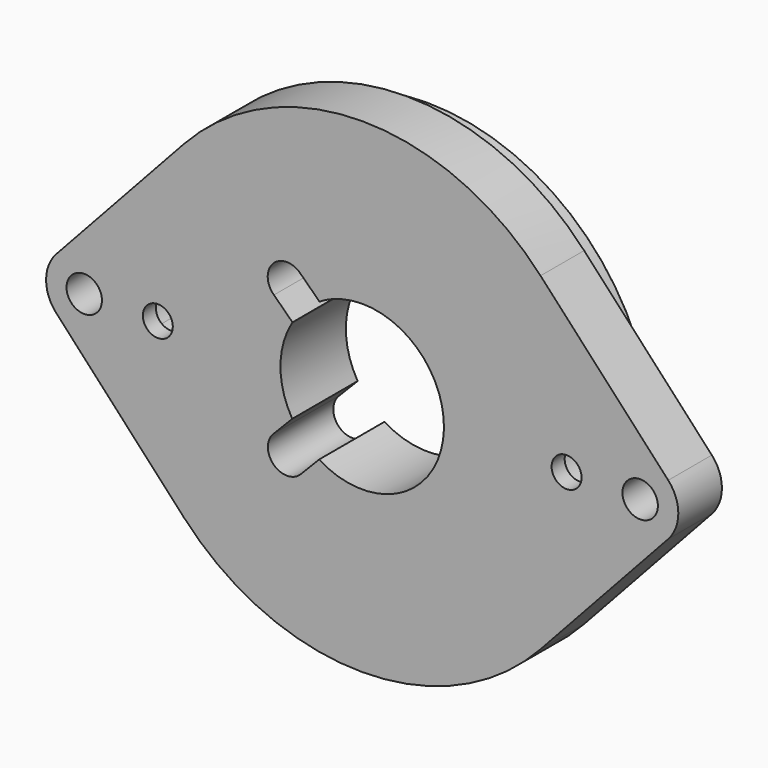
from build123d import *

# Parameters (mm, degrees)
F0_R        = 3.25
F0_R_2      = 41.5
F0_R_3      = 2.75
F1_DEPTH    = 10
F2_DEPTH    = 15
F3_R        = 2.75
F4_DEPTH    = 12
F5_T2_ANGLE = 170.4527374882
F5_T4_ANGLE = 170.4527374882


# Not quite as in the source:
# - a fillet or chamfer that OpenCascade refuses, or shapes differently, is made with other operations: its cross-section is extruded or revolved along the edge and cut away or added


with BuildPart() as f1:
    # F0 (on Front) → F1 (new body)
    with BuildSketch(Plane.XZ):
        with BuildLine():
            Line((56.1470588235, 4.7442370796), (32.7205882353, 30.159792863))
            ThreePointArc((32.7205882353, 30.159792863), (0, 44.5), (-32.7205882353, 30.159792863))
            Line((-32.7205882353, 30.159792863), (-56.1470588235, 4.7442370796))
            ThreePointArc((-56.1470588235, 4.7442370796), (-58, 0), (-56.1470588235, -4.7442370796))
            Line((-56.1470588235, -4.7442370796), (-32.7205882353, -30.159792863))
            ThreePointArc((-32.7205882353, -30.159792863), (0, -44.5), (32.7205882353, -30.159792863))
            Line((32.7205882353, -30.159792863), (56.1470588235, -4.7442370796))
            ThreePointArc((56.1470588235, -4.7442370796), (58, 0), (56.1470588235, 4.7442370796))
        make_face()
        with Locations((-51, 0)):
            Circle(F0_R, mode=Mode.SUBTRACT)
        Circle(F0_R_2, mode=Mode.SUBTRACT)
        with Locations((51, 0)):
            Circle(F0_R, mode=Mode.SUBTRACT)
        Circle(F0_R_2)
        with BuildLine():
            ThreePointArc((-5.5275883623, 13.9443811945), (14.9403084329, -1.336855987), (-7.9154361587, -12.7415018902))
            Line((-7.9154361587, -12.7415018902), (-11.2935258895, -16.2148281895))
            ThreePointArc((-11.2935258895, -16.2148281895), (-16.2431437728, -16.28328537), (-16.3109133443, -11.3336580242))
            Line((-16.3109133443, -11.3336580242), (-12.8354378119, -7.7621863014))
            ThreePointArc((-12.8354378119, -7.7621863014), (-14.9994558699, -0.1277638746), (-12.9658008757, 7.5424139141))
            ThreePointArc((-12.9658008757, 7.5424139141), (-12.8781036996, 7.6911926971), (-12.7886994065, 7.8389519382))
            Line((-12.7886994065, 7.8389519382), (-16.1911722961, 11.1499710909))
            ThreePointArc((-16.1911722961, 11.1499710909), (-16.3869084591, 16.1374875976), (-11.3967981993, 16.2489916113))
            Line((-11.3967981993, 16.2489916113), (-7.8389519382, 12.7886994065))
            ThreePointArc((-7.8389519382, 12.7886994065), (-6.7082039325, 13.416407865), (-5.5275883623, 13.9443811945))
        make_face(mode=Mode.SUBTRACT)
        with Locations((-37.5, 0)):
            Circle(F0_R_3, mode=Mode.SUBTRACT)
        with Locations((37.5, 0)):
            Circle(F0_R_3, mode=Mode.SUBTRACT)
    extrude(amount=-F1_DEPTH)

    # F0 (on Front) → F2 (join)
    with BuildSketch(Plane.XZ):
        Circle(F0_R_2)
        with BuildLine():
            ThreePointArc((-5.5275883623, 13.9443811945), (14.9403084329, -1.336855987), (-7.9154361587, -12.7415018902))
            Line((-7.9154361587, -12.7415018902), (-11.2935258895, -16.2148281895))
            ThreePointArc((-11.2935258895, -16.2148281895), (-16.2431437728, -16.28328537), (-16.3109133443, -11.3336580242))
            Line((-16.3109133443, -11.3336580242), (-12.8354378119, -7.7621863014))
            ThreePointArc((-12.8354378119, -7.7621863014), (-14.9994558699, -0.1277638746), (-12.9658008757, 7.5424139141))
            ThreePointArc((-12.9658008757, 7.5424139141), (-12.8781036996, 7.6911926971), (-12.7886994065, 7.8389519382))
            Line((-12.7886994065, 7.8389519382), (-16.1911722961, 11.1499710909))
            ThreePointArc((-16.1911722961, 11.1499710909), (-16.3869084591, 16.1374875976), (-11.3967981993, 16.2489916113))
            Line((-11.3967981993, 16.2489916113), (-7.8389519382, 12.7886994065))
            ThreePointArc((-7.8389519382, 12.7886994065), (-6.7082039325, 13.416407865), (-5.5275883623, 13.9443811945))
        make_face(mode=Mode.SUBTRACT)
        with Locations((-37.5, 0)):
            Circle(F0_R_3, mode=Mode.SUBTRACT)
        with Locations((37.5, 0)):
            Circle(F0_R_3, mode=Mode.SUBTRACT)
    extrude(amount=-F2_DEPTH)

    # F3 (on face) → F4 (cut)
    with BuildSketch(Plane(origin=(0, 15, 0), x_dir=(-1, 0, 0), z_dir=(0, 1, 0))):
        with BuildLine():
            ThreePointArc((41.31, -3.9665980386), (42.5598913032, -2.1558061137), (43, 0))
            ThreePointArc((43, 0), (42.5598913032, 2.1558061137), (41.31, 3.9665980386))
            ThreePointArc((41.31, 3.9665980386), (41.4524727851, 1.9855729652), (41.5, 0))
            ThreePointArc((41.5, 0), (41.4524727851, -1.9855729652), (41.31, -3.9665980386))
        make_face()
        with BuildLine():
            ThreePointArc((41.5, 0), (41.4524727851, 1.9855729652), (41.31, 3.9665980386))
            ThreePointArc((41.31, 3.9665980386), (32, 0), (41.31, -3.9665980386))
            ThreePointArc((41.31, -3.9665980386), (41.4524727851, -1.9855729652), (41.5, 0))
        make_face()
        with Locations((37.5, 0)):
            Circle(F3_R, mode=Mode.SUBTRACT)
        with BuildLine():
            ThreePointArc((-41.31, -3.9665980386), (-41.5, 0), (-41.31, 3.9665980386))
            ThreePointArc((-41.31, 3.9665980386), (-43, 0), (-41.31, -3.9665980386))
        make_face()
        with BuildLine():
            ThreePointArc((-32, 0), (-35.3441938863, 5.0598913032), (-41.31, 3.9665980386))
            ThreePointArc((-41.31, 3.9665980386), (-41.5, 0), (-41.31, -3.9665980386))
            ThreePointArc((-41.31, -3.9665980386), (-35.3441938863, -5.0598913032), (-32, 0))
        make_face()
        with Locations((-37.5, 0)):
            Circle(F3_R, mode=Mode.SUBTRACT)
        with Locations((37.5, 0)):
            Circle(F3_R)
        with Locations((-37.5, 0)):
            Circle(F3_R)
    extrude(amount=-F4_DEPTH, mode=Mode.SUBTRACT)

    # F5: chamfer of 0.2 on 2 edges, made by hand

    # F5_s1 → F5_t2 (revolve, cut)
    with BuildSketch(Plane(origin=(0, 0, 0), x_dir=(0, 1, 0), z_dir=(0.0832192271, 0, -0.9965312641))):
        Polygon((14.8, 41.5), (15, 41.3), (15, 41.5), align=None)
    revolve(axis=Axis((0, 15, 0), (0, -1, 0)), revolution_arc=F5_T2_ANGLE, mode=Mode.SUBTRACT)

    # F5_s3 → F5_t4 (revolve, cut)
    with BuildSketch(Plane(origin=(0, 0, 0), x_dir=(0, 1, 0), z_dir=(-0.0832192271, 0, 0.9965312641))):
        Polygon((14.8, 41.5), (15, 41.3), (15, 41.5), align=None)
    revolve(axis=Axis((0, 15, 0), (0, -1, 0)), revolution_arc=F5_T4_ANGLE, mode=Mode.SUBTRACT)


solid = f1.part
